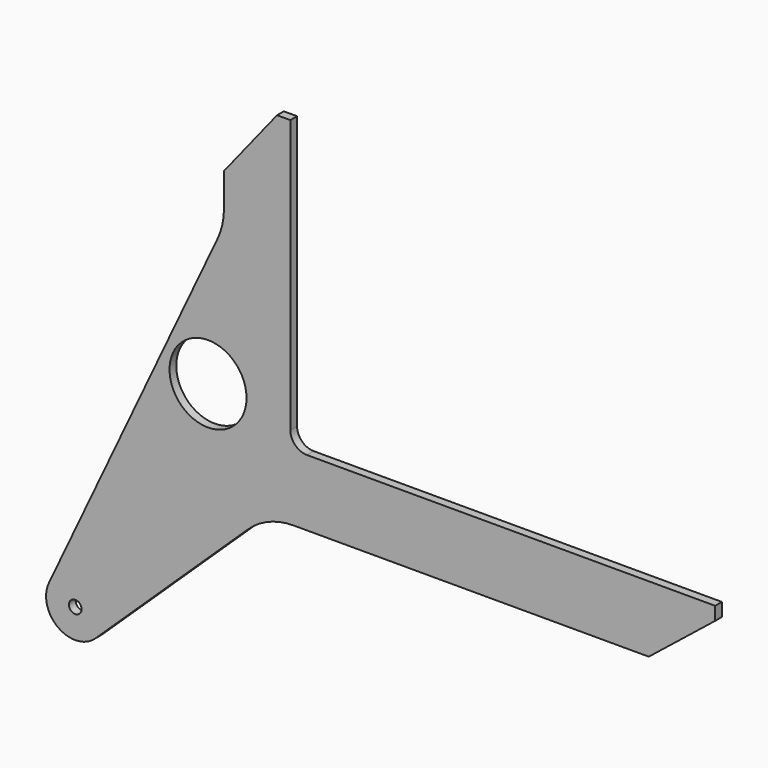
from build123d import *

# Parameters (mm, degrees)
F0_R     = 9.525
F0_R_2   = 58
F1_DEPTH = 6.35


# Not quite as in the source:
# - a feature names something its author has since deleted; it is built from what else it names


with BuildPart() as f1:
    # F0 (on Front) → F1 (new body, symmetric)
    with BuildSketch(Plane.XZ):
        with BuildLine():
            Line((14.4609105581, 197.3757855088), (-239.8028006456, -342.2453456239))
            ThreePointArc((-239.8028006456, -342.2453456239), (-225.7250673292, -396.6962310463), (-169.6171250668, -392.8257900262))
            Line((-169.6171250668, -392.8257900262), (59.9480115155, -173.6686590313))
            ThreePointArc((59.9480115155, -173.6686590313), (91.8054714835, -153.1745344831), (129, -146))
            Line((129, -146), (664, -146))
            Line((664, -146), (764, -66))
            Line((764, -66), (764, -46))
            Line((764, -46), (149, -46))
            ThreePointArc((149, -46), (131.3223304703, -38.6776695297), (124, -21))
            Line((124, -21), (124, 390))
            Line((124, 390), (104, 390))
            Line((104, 390), (24, 290))
            Line((24, 290), (24, 240))
            ThreePointArc((24, 240), (21.5860929022, 218.1607126469), (14.4609105581, 197.3757855088))
        make_face()
        with Locations((-200, -361)):
            Circle(F0_R, mode=Mode.SUBTRACT)
        Circle(F0_R_2, mode=Mode.SUBTRACT)
    extrude(amount=F1_DEPTH, both=True)


solid = f1.part
